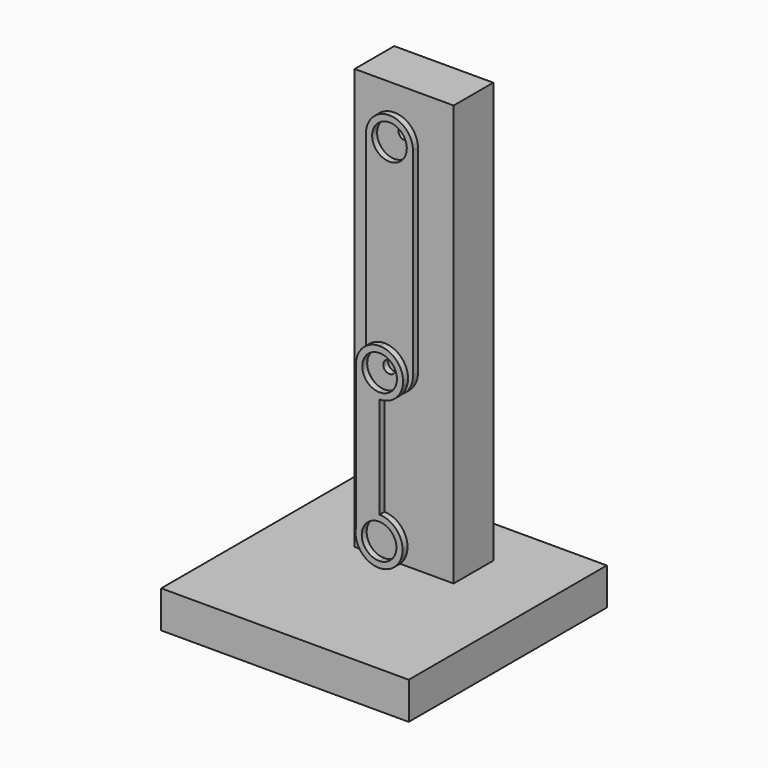
from build123d import *

# Parameters (mm, degrees)
F0_R      = 8.89
F0_R_2    = 3.175
F1_DEPTH  = 3.175
F4_DEPTH  = 3.175
F7_DEPTH  = 19.05
F9_DEPTH  = 215.9
F10_R     = 3.175
F11_DEPTH = 101.8252484294
F10_R_2   = 6.35
F12_DEPTH = 3.175


with BuildPart() as f1:
    # F0 (on Front) → F1 (new body)
    with BuildSketch(Plane.XZ):
        with BuildLine():
            ThreePointArc((-61.0184661174, 80.8981371284), (-48.9534661174, 68.8331371284), (-36.8884661174, 80.8981371284))
            ThreePointArc((-36.8884661174, 80.8981371284), (-48.9534661174, 92.9631371284), (-61.0184661174, 80.8981371284))
        make_face()
        with Locations((-48.9534661174, 80.8981371284)):
            Circle(F0_R, mode=Mode.SUBTRACT)
        with BuildLine():
            Line((-36.8884661174, -20.7018628716), (-36.8884661174, 80.8981371284))
            ThreePointArc((-36.8884661174, 80.8981371284), (-48.9534661174, 68.8331371284), (-61.0184661174, 80.8981371284))
            Line((-61.0184661174, 80.8981371284), (-61.0184661174, -20.7018628716))
            ThreePointArc((-61.0184661174, -20.7018628716), (-48.9534661174, -8.6368628716), (-36.8884661174, -20.7018628716))
        make_face()
        with BuildLine():
            ThreePointArc((-61.0184661174, -20.7018628716), (-48.9534661174, -32.7668628716), (-36.8884661174, -20.7018628716))
            ThreePointArc((-36.8884661174, -20.7018628716), (-48.9534661174, -8.6368628716), (-61.0184661174, -20.7018628716))
        make_face()
        with Locations((-48.9534661174, -20.7018628716)):
            Circle(F0_R_2, mode=Mode.SUBTRACT)
    extrude(amount=F1_DEPTH)


with BuildPart() as f4:
    # F3 (on offset) → F4 (new body)
    with BuildSketch(Plane.XZ.offset(6.35)):
        with BuildLine():
            Line((-48.9942056675, -84.8389475658), (-48.9942056675, -32.7667940894))
            ThreePointArc((-48.9942056675, -32.7667940894), (-57.4991008999, -29.218690401), (-61.0184661174, -20.7018628716))
            Line((-61.0184661174, -20.7018628716), (-61.0184661174, -94.3869631738))
            ThreePointArc((-61.0184661174, -94.3869631738), (-56.7211762043, -87.453377151), (-48.9942056675, -84.8389475658))
        make_face()
        with BuildLine():
            ThreePointArc((-48.9942056675, -29.5917695241), (-57.8434661174, -20.7018628716), (-48.9942056675, -11.8119562192))
            Line((-48.9942056675, -11.8119562192), (-48.9942056675, -8.6369316539))
            ThreePointArc((-48.9942056675, -8.6369316539), (-57.4991008999, -12.1850353423), (-61.0184661174, -20.7018628716))
            ThreePointArc((-61.0184661174, -20.7018628716), (-57.4991008999, -29.218690401), (-48.9942056675, -32.7667940894))
            Line((-48.9942056675, -32.7667940894), (-48.9942056675, -29.5917695241))
        make_face()
        with BuildLine():
            Line((-48.9942056675, -8.6369316539), (-48.9942056675, -11.8119562192))
            ThreePointArc((-48.9942056675, -11.8119562192), (-42.6817069782, -14.4012964447), (-40.0634661174, -20.7018628716))
            ThreePointArc((-40.0634661174, -20.7018628716), (-42.6817069782, -27.0024292986), (-48.9942056675, -29.5917695241))
            Line((-48.9942056675, -29.5917695241), (-48.9942056675, -32.7667940894))
            ThreePointArc((-48.9942056675, -32.7667940894), (-41.3791205839, -30.0930030974), (-37.1534868789, -23.2167614721))
            ThreePointArc((-37.1534868789, -23.2167614721), (-36.9549042345, -21.9662748866), (-36.8884661174, -20.7018628716))
            ThreePointArc((-36.8884661174, -20.7018628716), (-40.4366385881, -12.1562280891), (-48.9942056675, -8.6369316539))
        make_face()
        with BuildLine():
            Line((-48.9942056675, -88.0146923465), (-48.9942056675, -84.8389475658))
            ThreePointArc((-48.9942056675, -84.8389475658), (-56.7211762043, -87.453377151), (-61.0184661174, -94.3869631738))
            ThreePointArc((-61.0184661174, -94.3869631738), (-58.5258694104, -104.5788974785), (-48.9942056675, -108.9647781775))
            Line((-48.9942056675, -108.9647781775), (-48.9942056675, -105.7890333968))
            ThreePointArc((-48.9942056675, -105.7890333968), (-58.1084871101, -96.9018628716), (-48.9942056675, -88.0146923465))
        make_face()
        with BuildLine():
            ThreePointArc((-37.1534868789, -96.9018628716), (-40.6083133021, -88.450286878), (-48.9942056675, -84.8389475658))
            Line((-48.9942056675, -84.8389475658), (-48.9942056675, -88.0146923465))
            ThreePointArc((-48.9942056675, -88.0146923465), (-42.8535061195, -90.6954854648), (-40.3284868789, -96.9018628716))
            ThreePointArc((-40.3284868789, -96.9018628716), (-42.8535061195, -103.1082402785), (-48.9942056675, -105.7890333968))
            Line((-48.9942056675, -105.7890333968), (-48.9942056675, -108.9647781775))
            ThreePointArc((-48.9942056675, -108.9647781775), (-40.6083133021, -105.3534388653), (-37.1534868789, -96.9018628716))
        make_face()
    extrude(amount=F4_DEPTH)


with BuildPart() as f7:
    # F6 (on offset) → F7 (new body)
    with BuildSketch(Plane.XY.offset(-114.3)):
        Polygon((14.2815130055, -69.85), (14.2815130055, 57.15), (-49.2184869945, 57.15), (-112.7184869945, 57.15), (-112.7184869945, -69.85), align=None)
    extrude(amount=-F7_DEPTH)

    # F8 (on offset) → F9 (join)
    with BuildSketch(Plane.XY.offset(-114.3)):
        Polygon((-74.6184869945, 6.5742484294), (-49.2184869945, 6.5742484294), (-23.8184869945, 6.5742484294), (-23.8184869945, 31.9742484294), (-74.6184869945, 31.9742484294), align=None)
    extrude(amount=F9_DEPTH)

    # F10 (on face) → F11 (cut, through all)
    with BuildSketch(Plane(origin=(0, 31.9742484294, 0), x_dir=(-1, 0, 0), z_dir=(0, 1, 0))):
        with Locations((48.9534661174, 80.8981371284)):
            Circle(F10_R)
    extrude(amount=-F11_DEPTH, mode=Mode.SUBTRACT)

    # F10 (on face) → F12 (cut)
    with BuildSketch(Plane(origin=(0, 31.9742484294, 0), x_dir=(-1, 0, 0), z_dir=(0, 1, 0))):
        with Locations((48.9534661174, 80.8981371284)):
            Circle(F10_R_2)
        with Locations((48.9534661174, 80.8981371284)):
            Circle(F10_R, mode=Mode.SUBTRACT)
        with Locations((48.9534661174, 80.8981371284)):
            Circle(F10_R)
    extrude(amount=-F12_DEPTH, mode=Mode.SUBTRACT)


solid = Compound([f1.part, f4.part, f7.part])
